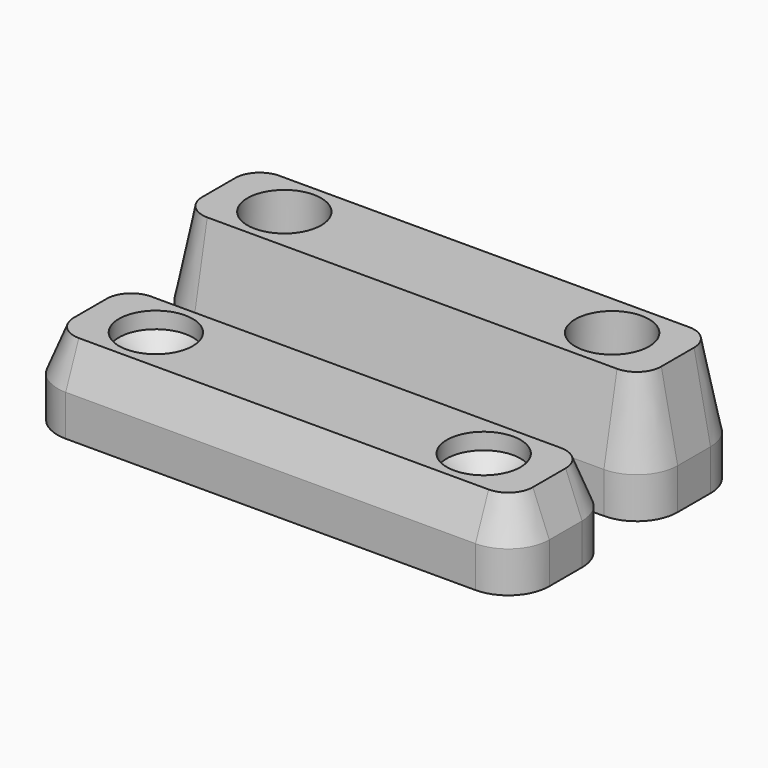
from build123d import *

# Parameters (mm, degrees)
F0_R      = 4.5
F1_DEPTH  = 10
F0_R_2    = 2.5
F2_DEPTH  = 8
F3_SIZE2  = 2
F3_SIZE   = 5
F4_SIZE   = 1.99999
F4_2_SIZE = 1.99999
F4_3_SIZE = 1.99999
F5_DEPTH  = 15
F6_SIZE2  = 2
F6_SIZE   = 10


# Not quite as in the source:
# - a fillet or chamfer is up to 0.001 mm smaller than in the source, because OpenCascade refuses the exact size
# - a feature names something its author has since deleted; it is built from what else it names


with BuildPart() as f1:
    # F0 (on Top) → F1 (new body)
    with BuildSketch(Plane.XY):
        with BuildLine():
            Line((55, -26.7175590992), (5, -26.7175590992))
            ThreePointArc((5, -26.7175590992), (1.4644660941, -28.1820251933), (0, -31.7175590992))
            Line((0, -31.7175590992), (0, -36.7175590992))
            ThreePointArc((0, -36.7175590992), (1.4644660941, -40.2530930051), (5, -41.7175590992))
            Line((5, -41.7175590992), (55, -41.7175590992))
            ThreePointArc((55, -41.7175590992), (58.5355339059, -40.2530930051), (60, -36.7175590992))
            Line((60, -36.7175590992), (60, -31.7175590992))
            ThreePointArc((60, -31.7175590992), (58.5355339059, -28.1820251933), (55, -26.7175590992))
        make_face()
        with Locations((10, -34.2175590992)):
            Circle(F0_R, mode=Mode.SUBTRACT)
        with Locations((50, -34.2175590992)):
            Circle(F0_R, mode=Mode.SUBTRACT)
    extrude(amount=F1_DEPTH)

    # F0 (on Top) → F2 (join)
    with BuildSketch(Plane.XY):
        with Locations((50, -34.2175590992)):
            Circle(F0_R)
        with Locations((50, -34.2175590992)):
            Circle(F0_R_2, mode=Mode.SUBTRACT)
        with Locations((10, -34.2175590992)):
            Circle(F0_R)
        with Locations((10, -34.2175590992)):
            Circle(F0_R_2, mode=Mode.SUBTRACT)
    extrude(amount=F2_DEPTH)

    # F3
    f3_edges = [f1.edges().sort_by_distance(p)[0] for p in [
        (30, -26.717559, 10),
    ]]
    f3_side = f1.faces().sort_by_distance((30, -26.717559, 5))[0]
    chamfer(f3_edges, length=F3_SIZE, length2=F3_SIZE2, reference=f3_side)

    # F4 (size 2 in the source; OpenCascade refuses exactly that, so slightly less here)
    f4_edges = [f1.edges().sort_by_distance(p)[0] for p in [
        (47.5, -34.217559, 8),
        (7.5, -34.217559, 8),
    ]]
    chamfer(f4_edges, length=F4_SIZE)


with BuildPart() as f2:
    # F0 (on Top) → F2, piece 2 (new body)
    with BuildSketch(Plane.XY):
        with Locations((10, -14.6273694187)):
            Circle(F0_R)
        with Locations((10, -14.6273694187)):
            Circle(F0_R_2, mode=Mode.SUBTRACT)
    extrude(amount=F2_DEPTH)

    # F4#2 (size 2 in the source; OpenCascade refuses exactly that, so slightly less here)
    f4_2_edges = [f2.edges().sort_by_distance(p)[0] for p in [
        (7.5, -14.627369, 8),
    ]]
    chamfer(f4_2_edges, length=F4_2_SIZE)



with BuildPart() as f2b:
    # F0 (on Top) → F2, piece 3 (new body)
    with BuildSketch(Plane.XY):
        with Locations((50, -14.6273694187)):
            Circle(F0_R)
        with Locations((50, -14.6273694187)):
            Circle(F0_R_2, mode=Mode.SUBTRACT)
    extrude(amount=F2_DEPTH)

    # F4#3 (size 2 in the source; OpenCascade refuses exactly that, so slightly less here)
    f4_3_edges = [f2b.edges().sort_by_distance(p)[0] for p in [
        (47.5, -14.627369, 8),
    ]]
    chamfer(f4_3_edges, length=F4_3_SIZE)


with BuildPart() as f2_1:
    add(f2.part)

    add(f2b.part)  # F5 merges F2b
    # F0 (on Top) → F5 (join)
    with BuildSketch(Plane.XY):
        with BuildLine():
            Line((55, -7.1273694187), (5, -7.1273694187))
            ThreePointArc((5, -7.1273694187), (1.4644660941, -8.5918355128), (0, -12.1273694187))
            Line((0, -12.1273694187), (0, -17.1273694187))
            ThreePointArc((0, -17.1273694187), (1.4644660941, -20.6629033247), (5, -22.1273694187))
            Line((5, -22.1273694187), (55, -22.1273694187))
            ThreePointArc((55, -22.1273694187), (58.5355339059, -20.6629033247), (60, -17.1273694187))
            Line((60, -17.1273694187), (60, -12.1273694187))
            ThreePointArc((60, -12.1273694187), (58.5355339059, -8.5918355128), (55, -7.1273694187))
        make_face()
        with Locations((10, -14.6273694187)):
            Circle(F0_R, mode=Mode.SUBTRACT)
        with Locations((50, -14.6273694187)):
            Circle(F0_R, mode=Mode.SUBTRACT)
    extrude(amount=F5_DEPTH)

    # F6
    f6_edges = [f2_1.edges().sort_by_distance(p)[0] for p in [
        (30, -7.127369, 15),
    ]]
    f6_side = f2_1.faces().sort_by_distance((30, -7.127369, 7.5))[0]
    chamfer(f6_edges, length=F6_SIZE, length2=F6_SIZE2, reference=f6_side)


solid = Compound([f1.part, f2_1.part])
